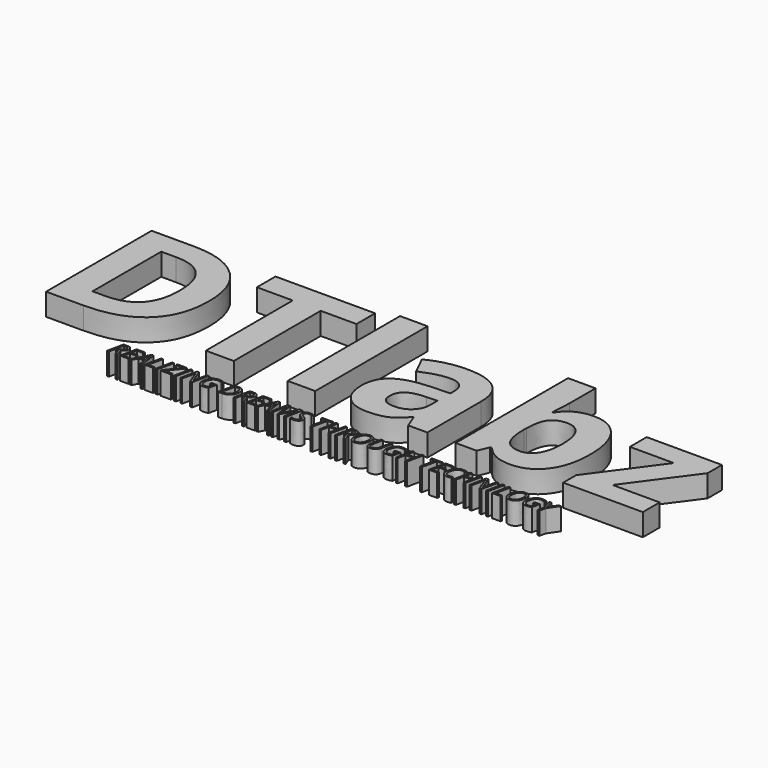
from build123d import *

# Parameters (mm, degrees)
F0_TEXT_SIZE   = 105.8333333333
F0_TEXT_SIZE_2 = 13.1880612998
F1_DEPTH       = 12.7


# Not quite as in the source:
# - Text() gives the source's letters only with a copy of the font that has no kerning and outlines rounded to 1/6400 em; it was checked with that copy


with BuildPart() as f1:
    # F0 (on Top) → F1 (new body)
    with BuildSketch(Plane.XY):
        with Locations((-195.0310850742, -9.481219139)):
            Text('DTlabz', F0_TEXT_SIZE, font='Open Sans', font_style=FontStyle.BOLD, text_align=(TextAlign.LEFT, TextAlign.BOTTOM))
        with Locations((-129.0338805794, -37.2029927371)):
            Text('REALIZING DREAMS THROUGH TECHNILOGY', F0_TEXT_SIZE_2, font='Open Sans', font_style=FontStyle.ITALIC, text_align=(TextAlign.LEFT, TextAlign.BOTTOM))
    extrude(amount=F1_DEPTH)


solid = f1.part
